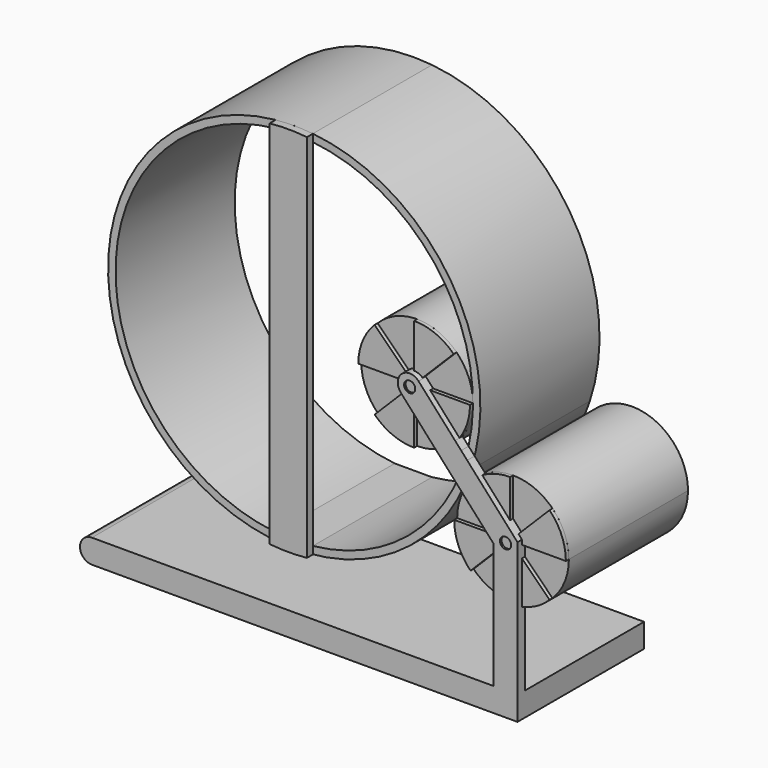
from build123d import *

# Parameters (mm, degrees)
F1_DEPTH  = 25
F2_DEPTH  = 400
F3_DEPTH  = 20
F4_DEPTH  = 500
F5_DEPTH  = 500
F6_DEPTH  = 400
F7_DEPTH  = 400
F8_DEPTH  = 20
F10_DEPTH = 10


with BuildPart() as f1:
    # F0 (on Front) → F1 (new body)
    with BuildSketch(Plane.XZ):
        with BuildLine():
            Line((619.5925408203, -698.0510845184), (619.5925408203, -634.0510845184))
            Line((619.5925408203, -634.0510845184), (587.5925408203, -634.0510845184))
            Line((587.5925408203, -634.0510845184), (555.5925408203, -634.0510845184))
            Line((555.5925408203, -634.0510845184), (-523.4671831131, -634.0510845184))
            ThreePointArc((-523.4671831131, -634.0510845184), (-555.4671831131, -666.0510845184), (-523.4671831131, -698.0510845184))
            Line((-523.4671831131, -698.0510845184), (619.5925408203, -698.0510845184))
        make_face()
        with BuildLine():
            Line((571.5025570686, -267.6097967695), (487.0976257639, -174.0804081495))
            ThreePointArc((487.0976257639, -174.0804081495), (475.7304372594, -185.5048345789), (465.6545376167, -198.0828606612))
            Line((465.6545376167, -198.0828606612), (555.5925408203, -297.7434648854))
            Line((555.5925408203, -297.7434648854), (555.5925408203, -431.9860827629))
            ThreePointArc((555.5925408203, -431.9860827629), (571.4996560892, -434.5733936367), (587.5925408203, -435.4391619491))
            Line((587.5925408203, -435.4391619491), (587.5925408203, -310.6819911327))
            Line((587.5925408203, -310.6819911327), (567.0049632483, -304.0182748497))
            Line((567.0049632483, -304.0182748497), (561.2087682826, -276.8993532197))
            Line((561.2087682826, -276.8993532197), (571.5025570686, -267.6097967695))
        make_face()
        with BuildLine():
            Line((619.5925408203, -273.1348590129), (513.1676059045, -155.2050302371))
            ThreePointArc((513.1676059045, -155.2050302371), (499.6248851086, -163.9414601248), (487.0976257639, -174.0804081495))
            Line((487.0976257639, -174.0804081495), (571.5025570686, -267.6097967695))
            Line((571.5025570686, -267.6097967695), (581.7963458546, -258.3202403192))
            Line((581.7963458546, -258.3202403192), (608.1801183922, -266.8600490486))
            Line((608.1801183922, -266.8600490486), (613.9763133579, -293.9789706786))
            Line((613.9763133579, -293.9789706786), (593.388735786, -312.5580835791))
            Line((593.388735786, -312.5580835791), (587.5925408203, -310.6819911327))
            Line((587.5925408203, -310.6819911327), (587.5925408203, -435.4391619491))
            ThreePointArc((587.5925408203, -435.4391619491), (603.6854255513, -434.5733936367), (619.5925408203, -431.9860827629))
            Line((619.5925408203, -431.9860827629), (619.5925408203, -273.1348590129))
        make_face()
        with BuildLine():
            Line((487.0976257639, -174.0804081495), (473.8942746161, -159.4497302791))
            ThreePointArc((473.8942746161, -159.4497302791), (467.8463381744, -176.4080606343), (461.1917687716, -193.1376514751))
            Line((461.1917687716, -193.1376514751), (465.6545376167, -198.0828606612))
            ThreePointArc((465.6545376167, -198.0828606612), (475.7304372594, -185.5048345789), (487.0976257639, -174.0804081495))
        make_face()
        with BuildLine():
            ThreePointArc((461.1917687716, -193.1376514751), (467.8463381744, -176.4080606343), (473.8942746161, -159.4497302791))
            Line((473.8942746161, -159.4497302791), (458.4208633436, -142.3035911399))
            ThreePointArc((458.4208633436, -142.3035911399), (452.692523658, -159.5916007319), (446.3124773798, -176.6498585765))
            Line((446.3124773798, -176.6498585765), (461.1917687716, -193.1376514751))
        make_face()
        with BuildLine():
            ThreePointArc((446.3124773798, -176.6498585765), (452.692523658, -159.5916007319), (458.4208633436, -142.3035911399))
            Line((458.4208633436, -142.3035911399), (430.4949150564, -111.3587537997))
            ThreePointArc((430.4949150564, -111.3587537997), (417.9676557116, -121.4977018244), (404.4249349157, -130.234131712))
            Line((404.4249349157, -130.234131712), (446.3124773798, -176.6498585765))
        make_face()
        with BuildLine():
            ThreePointArc((458.4208633436, -142.3035911399), (463.7127179959, -123.9778817726), (468.272302341, -105.4563931693))
            Line((468.272302341, -105.4563931693), (451.9380032036, -87.356301288))
            ThreePointArc((451.9380032036, -87.356301288), (441.8621035608, -99.9343273703), (430.4949150564, -111.3587537997))
            Line((430.4949150564, -111.3587537997), (458.4208633436, -142.3035911399))
        make_face()
        with BuildLine():
            ThreePointArc((430.4949150564, -111.3587537997), (441.8621035608, -99.9343273703), (451.9380032036, -87.356301288))
            Line((451.9380032036, -87.356301288), (353.7565341439, 21.438915212))
            ThreePointArc((353.7565341439, 21.438915212), (308.561084788, 23.7565341439), (306.2434658561, -21.438915212))
            Line((306.2434658561, -21.438915212), (404.4249349157, -130.234131712))
            ThreePointArc((404.4249349157, -130.234131712), (417.9676557116, -121.4977018244), (430.4949150564, -111.3587537997))
        make_face()
        Polygon((350.264825672, -16.1542842363), (346.0662299812, -17.8030435466), (326.1423923074, -25.6269959534), (305.8775666354, -9.4727117171), (309.735174328, 16.1542842363), (333.8576076926, 25.6269959534), (354.1224333646, 9.4727117171), align=None, mode=Mode.SUBTRACT)
        with BuildLine():
            ThreePointArc((473.8942746161, -159.4497302791), (479.5440529439, -141.553881212), (484.5182852707, -123.4586215636))
            Line((484.5182852707, -123.4586215636), (468.272302341, -105.4563931693))
            ThreePointArc((468.272302341, -105.4563931693), (463.7127179959, -123.9778817726), (458.4208633436, -142.3035911399))
            Line((458.4208633436, -142.3035911399), (473.8942746161, -159.4497302791))
        make_face()
        with BuildLine():
            Line((513.1676059045, -155.2050302371), (484.5182852707, -123.4586215636))
            ThreePointArc((484.5182852707, -123.4586215636), (479.5440529439, -141.553881212), (473.8942746161, -159.4497302791))
            Line((473.8942746161, -159.4497302791), (487.0976257639, -174.0804081495))
            ThreePointArc((487.0976257639, -174.0804081495), (499.6248851086, -163.9414601248), (513.1676059045, -155.2050302371))
        make_face()
        with BuildLine():
            Line((577.5430493146, -274.3032865692), (571.5025570686, -267.6097967695))
            Line((571.5025570686, -267.6097967695), (561.2087682826, -276.8993532197))
            Line((561.2087682826, -276.8993532197), (567.0049632483, -304.0182748497))
            Line((567.0049632483, -304.0182748497), (587.5925408203, -310.6819911327))
            Line((587.5925408203, -310.6819911327), (587.5925408203, -300.4391619491))
            ThreePointArc((587.5925408203, -300.4391619491), (573.5918599315, -290.822556292), (577.5430493146, -274.3032865692))
        make_face()
        with BuildLine():
            Line((581.7963458546, -258.3202403192), (571.5025570686, -267.6097967695))
            Line((571.5025570686, -267.6097967695), (577.5430493146, -274.3032865692))
            ThreePointArc((577.5430493146, -274.3032865692), (593.6858825724, -271.7325509058), (602.5925408203, -285.4391619491))
            ThreePointArc((602.5925408203, -285.4391619491), (598.1991425381, -296.0457636669), (587.5925408203, -300.4391619491))
            Line((587.5925408203, -300.4391619491), (587.5925408203, -310.6819911327))
            Line((587.5925408203, -310.6819911327), (593.388735786, -312.5580835791))
            Line((593.388735786, -312.5580835791), (613.9763133579, -293.9789706786))
            Line((613.9763133579, -293.9789706786), (608.1801183922, -266.8600490486))
            Line((608.1801183922, -266.8600490486), (581.7963458546, -258.3202403192))
        make_face()
        Polygon((326.1423923074, -25.6269959534), (346.0662299812, -17.8030435466), (350.264825672, -16.1542842363), (354.1224333646, 9.4727117171), (333.8576076926, 25.6269959534), (309.735174328, 16.1542842363), (305.8775666354, -9.4727117171), align=None)
        with BuildLine():
            ThreePointArc((345, 0), (343.7066110433, -6.0933417521), (340.0494915056, -11.13587538))
            ThreePointArc((340.0494915056, -11.13587538), (316.2933889567, 6.0933417521), (345, 0))
        make_face(mode=Mode.SUBTRACT)
        with BuildLine():
            ThreePointArc((587.5925408203, -435.4391619491), (571.4996560892, -434.5733936367), (555.5925408203, -431.9860827629))
            Line((555.5925408203, -431.9860827629), (555.5925408203, -634.0510845184))
            Line((555.5925408203, -634.0510845184), (587.5925408203, -634.0510845184))
            Line((587.5925408203, -634.0510845184), (587.5925408203, -435.4391619491))
        make_face()
        with BuildLine():
            Line((619.5925408203, -634.0510845184), (619.5925408203, -431.9860827629))
            ThreePointArc((619.5925408203, -431.9860827629), (603.6854255513, -434.5733936367), (587.5925408203, -435.4391619491))
            Line((587.5925408203, -435.4391619491), (587.5925408203, -634.0510845184))
            Line((587.5925408203, -634.0510845184), (619.5925408203, -634.0510845184))
        make_face()
    extrude(amount=F1_DEPTH)

    # F0 (on Front) → F2 (join)
    with BuildSketch(Plane.XZ):
        with BuildLine():
            Line((619.5925408203, -698.0510845184), (619.5925408203, -634.0510845184))
            Line((619.5925408203, -634.0510845184), (587.5925408203, -634.0510845184))
            Line((587.5925408203, -634.0510845184), (555.5925408203, -634.0510845184))
            Line((555.5925408203, -634.0510845184), (-523.4671831131, -634.0510845184))
            ThreePointArc((-523.4671831131, -634.0510845184), (-555.4671831131, -666.0510845184), (-523.4671831131, -698.0510845184))
            Line((-523.4671831131, -698.0510845184), (619.5925408203, -698.0510845184))
        make_face()
    extrude(amount=-F2_DEPTH)


with BuildPart() as f3:
    # F0 (on Front) → F3 (new body)
    with BuildSketch(Plane.XZ):
        Polygon((326.1423923074, -25.6269959534), (346.0662299812, -17.8030435466), (350.264825672, -16.1542842363), (354.1224333646, 9.4727117171), (333.8576076926, 25.6269959534), (309.735174328, 16.1542842363), (305.8775666354, -9.4727117171), align=None)
        with BuildLine():
            ThreePointArc((345, 0), (343.7066110433, -6.0933417521), (340.0494915056, -11.13587538))
            ThreePointArc((340.0494915056, -11.13587538), (316.2933889567, 6.0933417521), (345, 0))
        make_face(mode=Mode.SUBTRACT)
        with BuildLine():
            ThreePointArc((345, 0), (316.2933889567, 6.0933417521), (340.0494915056, -11.13587538))
            ThreePointArc((340.0494915056, -11.13587538), (343.7066110433, -6.0933417521), (345, 0))
        make_face()
    extrude(amount=F3_DEPTH)

    # F0 (on Front) → F4 (join)
    with BuildSketch(Plane.XZ):
        with BuildLine():
            ThreePointArc((345, 0), (316.2933889567, 6.0933417521), (340.0494915056, -11.13587538))
            ThreePointArc((340.0494915056, -11.13587538), (343.7066110433, -6.0933417521), (345, 0))
        make_face()
    extrude(amount=-F4_DEPTH)


with BuildPart() as f3b:
    # F0 (on Front) → F3, piece 2 (new body)
    with BuildSketch(Plane.XZ):
        with BuildLine():
            Line((577.5430493146, -274.3032865692), (571.5025570686, -267.6097967695))
            Line((571.5025570686, -267.6097967695), (561.2087682826, -276.8993532197))
            Line((561.2087682826, -276.8993532197), (567.0049632483, -304.0182748497))
            Line((567.0049632483, -304.0182748497), (587.5925408203, -310.6819911327))
            Line((587.5925408203, -310.6819911327), (587.5925408203, -300.4391619491))
            ThreePointArc((587.5925408203, -300.4391619491), (573.5918599315, -290.822556292), (577.5430493146, -274.3032865692))
        make_face()
        with BuildLine():
            Line((581.7963458546, -258.3202403192), (571.5025570686, -267.6097967695))
            Line((571.5025570686, -267.6097967695), (577.5430493146, -274.3032865692))
            ThreePointArc((577.5430493146, -274.3032865692), (593.6858825724, -271.7325509058), (602.5925408203, -285.4391619491))
            ThreePointArc((602.5925408203, -285.4391619491), (598.1991425381, -296.0457636669), (587.5925408203, -300.4391619491))
            Line((587.5925408203, -300.4391619491), (587.5925408203, -310.6819911327))
            Line((587.5925408203, -310.6819911327), (593.388735786, -312.5580835791))
            Line((593.388735786, -312.5580835791), (613.9763133579, -293.9789706786))
            Line((613.9763133579, -293.9789706786), (608.1801183922, -266.8600490486))
            Line((608.1801183922, -266.8600490486), (581.7963458546, -258.3202403192))
        make_face()
        with BuildLine():
            ThreePointArc((602.5925408203, -285.4391619491), (593.6858825724, -271.7325509058), (577.5430493146, -274.3032865692))
            Line((577.5430493146, -274.3032865692), (587.5925408203, -285.4391619491))
            Line((587.5925408203, -285.4391619491), (587.5925408203, -300.4391619491))
            ThreePointArc((587.5925408203, -300.4391619491), (598.1991425381, -296.0457636669), (602.5925408203, -285.4391619491))
        make_face()
        with BuildLine():
            Line((587.5925408203, -285.4391619491), (577.5430493146, -274.3032865692))
            ThreePointArc((577.5430493146, -274.3032865692), (573.5918599315, -290.822556292), (587.5925408203, -300.4391619491))
            Line((587.5925408203, -300.4391619491), (587.5925408203, -285.4391619491))
        make_face()
    extrude(amount=F3_DEPTH)

    # F0 (on Front) → F5 (join)
    with BuildSketch(Plane.XZ):
        with BuildLine():
            ThreePointArc((602.5925408203, -285.4391619491), (593.6858825724, -271.7325509058), (577.5430493146, -274.3032865692))
            Line((577.5430493146, -274.3032865692), (587.5925408203, -285.4391619491))
            Line((587.5925408203, -285.4391619491), (587.5925408203, -300.4391619491))
            ThreePointArc((587.5925408203, -300.4391619491), (598.1991425381, -296.0457636669), (602.5925408203, -285.4391619491))
        make_face()
        with BuildLine():
            Line((587.5925408203, -285.4391619491), (577.5430493146, -274.3032865692))
            ThreePointArc((577.5430493146, -274.3032865692), (573.5918599315, -290.822556292), (587.5925408203, -300.4391619491))
            Line((587.5925408203, -300.4391619491), (587.5925408203, -285.4391619491))
        make_face()
    extrude(amount=-F5_DEPTH)


with BuildPart() as f6:
    # F0 (on Front) → F6 (new body)
    with BuildSketch(Plane.XZ):
        with BuildLine():
            ThreePointArc((737.5925408203, -285.4391619491), (662.879524299, -155.7014645799), (513.1676059045, -155.2050302371))
            Line((513.1676059045, -155.2050302371), (619.5925408203, -273.1348590129))
            Line((619.5925408203, -273.1348590129), (619.5925408203, -431.9860827629))
            ThreePointArc((619.5925408203, -431.9860827629), (704.4257552757, -379.5136005603), (737.5925408203, -285.4391619491))
        make_face()
        with BuildLine():
            Line((619.5925408203, -273.1348590129), (513.1676059045, -155.2050302371))
            ThreePointArc((513.1676059045, -155.2050302371), (499.6248851086, -163.9414601248), (487.0976257639, -174.0804081495))
            Line((487.0976257639, -174.0804081495), (571.5025570686, -267.6097967695))
            Line((571.5025570686, -267.6097967695), (581.7963458546, -258.3202403192))
            Line((581.7963458546, -258.3202403192), (608.1801183922, -266.8600490486))
            Line((608.1801183922, -266.8600490486), (613.9763133579, -293.9789706786))
            Line((613.9763133579, -293.9789706786), (593.388735786, -312.5580835791))
            Line((593.388735786, -312.5580835791), (587.5925408203, -310.6819911327))
            Line((587.5925408203, -310.6819911327), (587.5925408203, -435.4391619491))
            ThreePointArc((587.5925408203, -435.4391619491), (603.6854255513, -434.5733936367), (619.5925408203, -431.9860827629))
            Line((619.5925408203, -431.9860827629), (619.5925408203, -273.1348590129))
        make_face()
        with BuildLine():
            Line((571.5025570686, -267.6097967695), (487.0976257639, -174.0804081495))
            ThreePointArc((487.0976257639, -174.0804081495), (475.7304372594, -185.5048345789), (465.6545376167, -198.0828606612))
            Line((465.6545376167, -198.0828606612), (555.5925408203, -297.7434648854))
            Line((555.5925408203, -297.7434648854), (555.5925408203, -431.9860827629))
            ThreePointArc((555.5925408203, -431.9860827629), (571.4996560892, -434.5733936367), (587.5925408203, -435.4391619491))
            Line((587.5925408203, -435.4391619491), (587.5925408203, -310.6819911327))
            Line((587.5925408203, -310.6819911327), (567.0049632483, -304.0182748497))
            Line((567.0049632483, -304.0182748497), (561.2087682826, -276.8993532197))
            Line((561.2087682826, -276.8993532197), (571.5025570686, -267.6097967695))
        make_face()
        with BuildLine():
            Line((555.5925408203, -297.7434648854), (465.6545376167, -198.0828606612))
            ThreePointArc((465.6545376167, -198.0828606612), (447.5857319324, -339.2731053773), (555.5925408203, -431.9860827629))
            Line((555.5925408203, -431.9860827629), (555.5925408203, -297.7434648854))
        make_face()
        with BuildLine():
            Line((577.5430493146, -274.3032865692), (571.5025570686, -267.6097967695))
            Line((571.5025570686, -267.6097967695), (561.2087682826, -276.8993532197))
            Line((561.2087682826, -276.8993532197), (567.0049632483, -304.0182748497))
            Line((567.0049632483, -304.0182748497), (587.5925408203, -310.6819911327))
            Line((587.5925408203, -310.6819911327), (587.5925408203, -300.4391619491))
            ThreePointArc((587.5925408203, -300.4391619491), (573.5918599315, -290.822556292), (577.5430493146, -274.3032865692))
        make_face()
        with BuildLine():
            Line((581.7963458546, -258.3202403192), (571.5025570686, -267.6097967695))
            Line((571.5025570686, -267.6097967695), (577.5430493146, -274.3032865692))
            ThreePointArc((577.5430493146, -274.3032865692), (593.6858825724, -271.7325509058), (602.5925408203, -285.4391619491))
            ThreePointArc((602.5925408203, -285.4391619491), (598.1991425381, -296.0457636669), (587.5925408203, -300.4391619491))
            Line((587.5925408203, -300.4391619491), (587.5925408203, -310.6819911327))
            Line((587.5925408203, -310.6819911327), (593.388735786, -312.5580835791))
            Line((593.388735786, -312.5580835791), (613.9763133579, -293.9789706786))
            Line((613.9763133579, -293.9789706786), (608.1801183922, -266.8600490486))
            Line((608.1801183922, -266.8600490486), (581.7963458546, -258.3202403192))
        make_face()
    extrude(amount=-F6_DEPTH)


with BuildPart() as f6b:
    # F0 (on Front) → F6, piece 2 (new body)
    with BuildSketch(Plane.XZ):
        with BuildLine():
            ThreePointArc((451.9380032036, -87.356301288), (472.8122902284, -45.8764619356), (480, 0))
            ThreePointArc((480, 0), (200.2623026307, 75.2869834787), (404.4249349157, -130.234131712))
            Line((404.4249349157, -130.234131712), (306.2434658561, -21.438915212))
            ThreePointArc((306.2434658561, -21.438915212), (308.561084788, 23.7565341439), (353.7565341439, 21.438915212))
            Line((353.7565341439, 21.438915212), (451.9380032036, -87.356301288))
        make_face()
        with BuildLine():
            ThreePointArc((430.4949150564, -111.3587537997), (441.8621035608, -99.9343273703), (451.9380032036, -87.356301288))
            Line((451.9380032036, -87.356301288), (353.7565341439, 21.438915212))
            ThreePointArc((353.7565341439, 21.438915212), (308.561084788, 23.7565341439), (306.2434658561, -21.438915212))
            Line((306.2434658561, -21.438915212), (404.4249349157, -130.234131712))
            ThreePointArc((404.4249349157, -130.234131712), (417.9676557116, -121.4977018244), (430.4949150564, -111.3587537997))
        make_face()
        Polygon((350.264825672, -16.1542842363), (346.0662299812, -17.8030435466), (326.1423923074, -25.6269959534), (305.8775666354, -9.4727117171), (309.735174328, 16.1542842363), (333.8576076926, 25.6269959534), (354.1224333646, 9.4727117171), align=None, mode=Mode.SUBTRACT)
        Polygon((326.1423923074, -25.6269959534), (346.0662299812, -17.8030435466), (350.264825672, -16.1542842363), (354.1224333646, 9.4727117171), (333.8576076926, 25.6269959534), (309.735174328, 16.1542842363), (305.8775666354, -9.4727117171), align=None)
        with BuildLine():
            ThreePointArc((345, 0), (343.7066110433, -6.0933417521), (340.0494915056, -11.13587538))
            ThreePointArc((340.0494915056, -11.13587538), (316.2933889567, 6.0933417521), (345, 0))
        make_face(mode=Mode.SUBTRACT)
    extrude(amount=-F6_DEPTH)


with BuildPart() as f7:
    # F0 (on Front) → F7 (new body)
    with BuildSketch(Plane.XZ):
        with BuildLine():
            ThreePointArc((484.5182852707, -123.4586215636), (496.1144740054, -62.2127694475), (500, 0))
            ThreePointArc((500, 0), (370.8099243548, 335.410196625), (50, 497.4937185533))
            Line((50, 497.4937185533), (50, 477.3887304912))
            ThreePointArc((50, 477.3887304912), (356.6510900025, 321.2475680842), (480, 0))
            ThreePointArc((480, 0), (477.0590661143, -53.053250967), (468.272302341, -105.4563931693))
            Line((468.272302341, -105.4563931693), (484.5182852707, -123.4586215636))
        make_face()
        with BuildLine():
            ThreePointArc((473.8942746161, -159.4497302791), (479.5440529439, -141.553881212), (484.5182852707, -123.4586215636))
            Line((484.5182852707, -123.4586215636), (468.272302341, -105.4563931693))
            ThreePointArc((468.272302341, -105.4563931693), (463.7127179959, -123.9778817726), (458.4208633436, -142.3035911399))
            Line((458.4208633436, -142.3035911399), (473.8942746161, -159.4497302791))
        make_face()
        with BuildLine():
            ThreePointArc((461.1917687716, -193.1376514751), (467.8463381744, -176.4080606343), (473.8942746161, -159.4497302791))
            Line((473.8942746161, -159.4497302791), (458.4208633436, -142.3035911399))
            ThreePointArc((458.4208633436, -142.3035911399), (452.692523658, -159.5916007319), (446.3124773798, -176.6498585765))
            Line((446.3124773798, -176.6498585765), (461.1917687716, -193.1376514751))
        make_face()
        with BuildLine():
            ThreePointArc((50, -497.4937185533), (297.4683344606, -401.8862898796), (461.1917687716, -193.1376514751))
            Line((461.1917687716, -193.1376514751), (446.3124773798, -176.6498585765))
            ThreePointArc((446.3124773798, -176.6498585765), (290.1594149271, -382.3709114579), (50, -477.3887304912))
            Line((50, -477.3887304912), (50, -497.4937185533))
        make_face()
        with BuildLine():
            Line((50, 477.3887304912), (50, 497.4937185533))
            ThreePointArc((50, 497.4937185533), (0, 500), (-50, 497.4937185533))
            Line((-50, 497.4937185533), (-50, 477.3887304912))
            Line((-50, 477.3887304912), (50, 477.3887304912))
        make_face()
        with BuildLine():
            Line((-50, 477.3887304912), (-50, 497.4937185533))
            ThreePointArc((-50, 497.4937185533), (-500, 0), (-50, -497.4937185533))
            Line((-50, -497.4937185533), (-50, -477.3887304912))
            ThreePointArc((-50, -477.3887304912), (-480, 0), (-50, 477.3887304912))
        make_face()
        with BuildLine():
            Line((-50, -477.3887304912), (-50, -497.4937185533))
            ThreePointArc((-50, -497.4937185533), (0, -500), (50, -497.4937185533))
            Line((50, -497.4937185533), (50, -477.3887304912))
            Line((50, -477.3887304912), (-50, -477.3887304912))
        make_face()
    extrude(amount=-F7_DEPTH)


with BuildPart() as f8:
    # F0 (on Front) → F8 (new body)
    with BuildSketch(Plane.XZ):
        Polygon((50, 0), (50, 477.3887304912), (-50, 477.3887304912), (-50, 0), (-50, -477.3887304912), (50, -477.3887304912), align=None)
        with BuildLine():
            Line((50, 477.3887304912), (50, 497.4937185533))
            ThreePointArc((50, 497.4937185533), (0, 500), (-50, 497.4937185533))
            Line((-50, 497.4937185533), (-50, 477.3887304912))
            Line((-50, 477.3887304912), (50, 477.3887304912))
        make_face()
        with BuildLine():
            Line((-50, -477.3887304912), (-50, -497.4937185533))
            ThreePointArc((-50, -497.4937185533), (0, -500), (50, -497.4937185533))
            Line((50, -497.4937185533), (50, -477.3887304912))
            Line((50, -477.3887304912), (-50, -477.3887304912))
        make_face()
    extrude(amount=F8_DEPTH)


with BuildPart() as f10:
    # F9 (on face) → F10 (new body)
    with BuildSketch(Plane.XZ):
        with BuildLine():
            ThreePointArc((223.933982822, -106.066017178), (272.5974851452, -138.5819298767), (330, -150))
            Line((330, -150), (330, -15))
            ThreePointArc((330, -15), (324.2597485145, -13.8581929877), (319.3933982822, -10.6066017178))
            Line((319.3933982822, -10.6066017178), (223.933982822, -106.066017178))
        make_face()
    extrude(amount=F10_DEPTH)


with BuildPart() as f10b:
    # F9 (on face) → F10, piece 2 (new body)
    with BuildSketch(Plane.XZ):
        with BuildLine():
            Line((319.3933982822, 10.6066017178), (223.933982822, 106.066017178))
            ThreePointArc((223.933982822, 106.066017178), (191.4180701233, 57.4025148548), (180, 0))
            Line((180, 0), (315, 0))
            ThreePointArc((315, 0), (316.1418070123, 5.7402514855), (319.3933982822, 10.6066017178))
        make_face()
    extrude(amount=F10_DEPTH)


with BuildPart() as f10c:
    # F9 (on face) → F10, piece 3 (new body)
    with BuildSketch(Plane.XZ):
        with BuildLine():
            Line((340.6066017178, 10.6066017178), (436.066017178, 106.066017178))
            ThreePointArc((436.066017178, 106.066017178), (387.4025148548, 138.5819298767), (330, 150))
            Line((330, 150), (330, 15))
            ThreePointArc((330, 15), (335.7402514855, 13.8581929877), (340.6066017178, 10.6066017178))
        make_face()
    extrude(amount=F10_DEPTH)


with BuildPart() as f10d:
    # F9 (on face) → F10, piece 4 (new body)
    with BuildSketch(Plane.XZ):
        with BuildLine():
            ThreePointArc((436.066017178, -106.066017178), (468.5819298767, -57.4025148548), (480, 0))
            Line((480, 0), (345, 0))
            ThreePointArc((345, 0), (343.8581929877, -5.7402514855), (340.6066017178, -10.6066017178))
            Line((340.6066017178, -10.6066017178), (436.066017178, -106.066017178))
        make_face()
    extrude(amount=F10_DEPTH)


with BuildPart() as f10e:
    # F9 (on face) → F10, piece 5 (new body)
    with BuildSketch(Plane.XZ):
        with BuildLine():
            Line((481.5265236423, -391.5051791271), (587.5925408203, -285.4391619491))
            Line((587.5925408203, -285.4391619491), (437.5925408203, -285.4391619491))
            ThreePointArc((437.5925408203, -285.4391619491), (449.0106109436, -342.8416768039), (481.5265236423, -391.5051791271))
        make_face()
    extrude(amount=F10_DEPTH)


with BuildPart() as f10f:
    # F9 (on face) → F10, piece 6 (new body)
    with BuildSketch(Plane.XZ):
        with BuildLine():
            Line((481.5265236423, -179.3731447712), (587.5925408203, -285.4391619491))
            Line((587.5925408203, -285.4391619491), (587.5925408203, -135.4391619491))
            ThreePointArc((587.5925408203, -135.4391619491), (530.1900259655, -146.8572320725), (481.5265236423, -179.3731447712))
        make_face()
    extrude(amount=F10_DEPTH)


with BuildPart() as f10g:
    # F9 (on face) → F10, piece 7 (new body)
    with BuildSketch(Plane.XZ):
        with BuildLine():
            Line((587.5925408203, -285.4391619491), (737.5925408203, -285.4391619491))
            ThreePointArc((737.5925408203, -285.4391619491), (726.174470697, -228.0366470944), (693.6585579983, -179.3731447712))
            Line((693.6585579983, -179.3731447712), (587.5925408203, -285.4391619491))
        make_face()
    extrude(amount=F10_DEPTH)


with BuildPart() as f10h:
    # F9 (on face) → F10, piece 8 (new body)
    with BuildSketch(Plane.XZ):
        with BuildLine():
            ThreePointArc((587.5925408203, -435.4391619491), (644.995055675, -424.0210918258), (693.6585579983, -391.5051791271))
            Line((693.6585579983, -391.5051791271), (587.5925408203, -285.4391619491))
            Line((587.5925408203, -285.4391619491), (587.5925408203, -435.4391619491))
        make_face()
    extrude(amount=F10_DEPTH)


solid = Compound([f1.part, f3.part, f3b.part, f6.part, f6b.part, f7.part, f8.part, f10.part, f10b.part, f10c.part, f10d.part, f10e.part, f10f.part, f10g.part, f10h.part])
